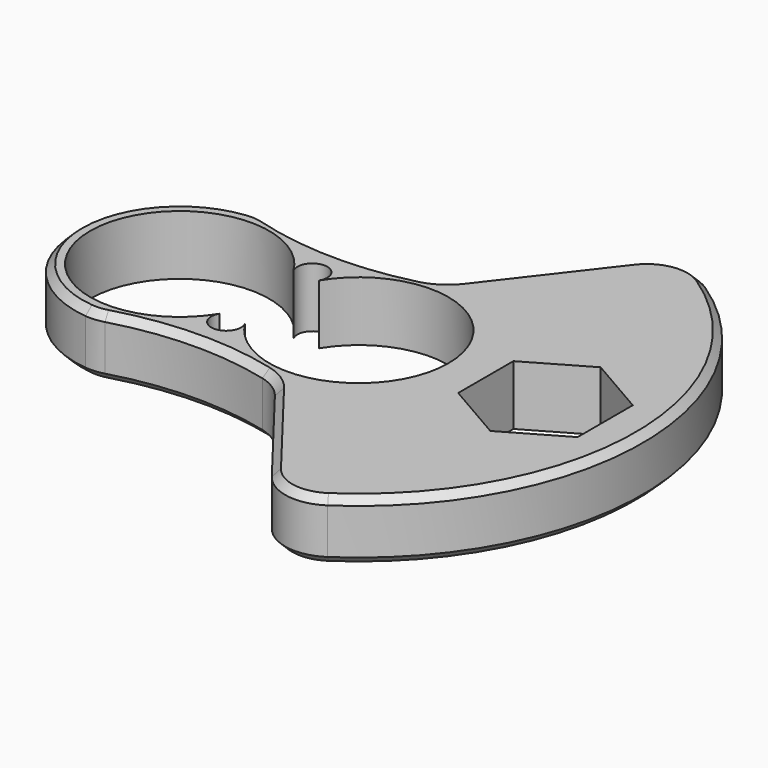
from build123d import *

# Parameters (mm, degrees)
F1_DEPTH = 6.35
F2_R     = 5.08
F3_SIZE  = 0.762


with BuildPart() as f1:
    # F0 (on Top) → F1 (new body)
    with BuildSketch(Plane.XY):
        with BuildLine():
            ThreePointArc((0, 11.1125), (-9.525, 9.650069645), (-19.05, 11.1125))
            ThreePointArc((-19.05, 11.1125), (-30.1625, 0), (-19.05, -11.1125))
            ThreePointArc((-19.05, -11.1125), (-9.525, -9.650069645), (0, -11.1125))
            Line((0, -11.1125), (12.5760834642, -27.4156621469))
            ThreePointArc((12.5760834642, -27.4156621469), (30.1625, 0), (12.5760834642, 27.4156621469))
            Line((12.5760834642, 27.4156621469), (0, 11.1125))
        make_face()
        Polygon((19.84375, -7.3323484187), (13.49375, -3.6661742094), (13.49375, 3.6661742094), (19.84375, 7.3323484187), (26.19375, 3.6661742094), (26.19375, -3.6661742094), align=None, mode=Mode.SUBTRACT)
        with BuildLine():
            ThreePointArc((-8.1642857143, 4.9061251284), (9.525, 0), (-8.1642857143, -4.9061251284))
            ThreePointArc((-8.1642857143, -4.9061251284), (-9.525, -7.3113126498), (-10.8857142857, -4.9061251284))
            ThreePointArc((-10.8857142857, -4.9061251284), (-28.575, 0), (-10.8857142857, 4.9061251284))
            ThreePointArc((-10.8857142857, 4.9061251284), (-9.525, 7.3113126498), (-8.1642857143, 4.9061251284))
        make_face(mode=Mode.SUBTRACT)
    extrude(amount=F1_DEPTH)

    # F2
    f2_edges = [f1.edges().sort_by_distance(p)[0] for p in [
        (12.576083, 27.415662, 3.175),
        (0, 11.1125, 3.175),
        (-19.05, 11.1125, 3.175),
        (-19.05, -11.1125, 3.175),
        (0, -11.1125, 3.175),
        (12.576083, -27.415662, 3.175),
    ]]
    fillet(f2_edges, radius=F2_R)

    # F3
    f3_edges = [f1.edges().sort_by_distance(p)[0] for p in [
        (30.1625, 0, 6.35),
        (30.1625, 0, 0),
        (5.466288, 18.198791, 0),
        (5.466288, 18.198791, 6.35),
        (13.111177, 25.870157, 0),
        (-0.214116, 11.292614, 0),
        (-10.037859, 9.654212, 0),
        (13.111177, -25.870157, 0),
        (-19.242874, 11.059803, 0),
        (5.466288, -18.198791, 0),
        (-30.1625, 0, 0),
        (-0.214116, -11.292614, 0),
        (-19.242874, -11.059803, 0),
        (-10.037859, -9.654212, 0),
        (13.111177, 25.870157, 6.35),
        (-0.214116, 11.292614, 6.35),
        (-10.037859, 9.654212, 6.35),
        (13.111177, -25.870157, 6.35),
        (-19.242874, 11.059803, 6.35),
        (5.466288, -18.198791, 6.35),
        (-30.1625, 0, 6.35),
        (-0.214116, -11.292614, 6.35),
        (-19.242874, -11.059803, 6.35),
        (-10.037859, -9.654212, 6.35),
    ]]
    chamfer(f3_edges, length=F3_SIZE)


solid = f1.part
